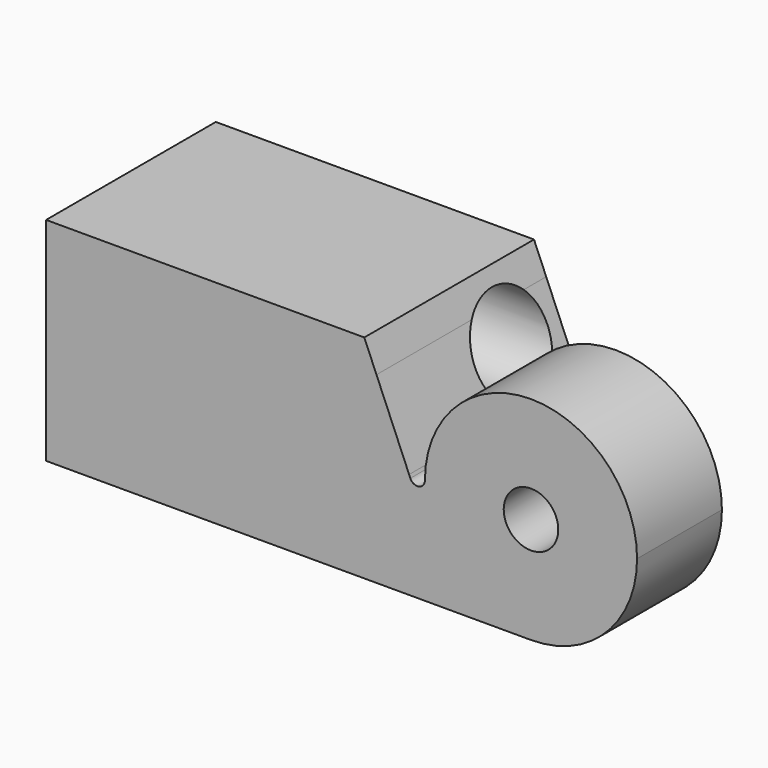
from build123d import *

# Parameters (mm, degrees)
F1_DEPTH       = 7
F2_D           = 3.6
F3_DEPTH       = 7
F5_D           = 3.5
F5_START       = 3.577541
F5_CBORE_D     = 6
F5_CBORE_DEPTH = 6


with BuildPart() as f1:
    # F0 (on Front) → F1 (new body)
    with BuildSketch(Plane.XZ):
        with BuildLine():
            Line((0, -7), (0, -1.45688))
            ThreePointArc((0, -1.45688), (-0.092433, -0.905477), (-0.1415, -0.348537))
            ThreePointArc((-0.1415, -0.348537), (-0.592364, -0.491395), (-0.960586, -0.194579))
            Line((-0.960586, -0.194579), (-1.042787, 0))
            Line((-1.042787, 0), (-3.195953, 5.096746))
            Line((-3.195953, 5.096746), (-4, 7))
            Line((-4, 7), (-25, 7))
            Line((-25, 7), (-25, -7))
            Line((-25, -7), (0, -7))
        make_face()
        with BuildLine():
            ThreePointArc((5.54312, -7), (1.944187, -5.055813), (0, -1.45688))
            Line((0, -1.45688), (0, -7))
            Line((0, -7), (5.54312, -7))
        make_face()
        with BuildLine():
            ThreePointArc((-0.1415, -0.348537), (-0.092433, -0.905477), (0, -1.45688))
            ThreePointArc((0, -1.45688), (1.944187, -5.055813), (5.54312, -7))
            Line((5.54312, -7), (7, -7))
            ThreePointArc((7, -7), (2.050253, -4.949747), (0, 0))
            ThreePointArc((0, 0), (-0.036724, -0.188082), (-0.1415, -0.348537))
        make_face()
        with BuildLine():
            ThreePointArc((14, 0), (7, 7), (0, 0))
            ThreePointArc((0, 0), (2.050253, -4.949747), (7, -7))
            ThreePointArc((7, -7), (11.949747, -4.949747), (14, 0))
        make_face()
    extrude(amount=F1_DEPTH)

    # F2 (through all)
    with Locations(Plane(origin=(0, 0, 0), x_dir=(1, 0, 0), z_dir=(0, 1, 0))):
        with Locations((7, 0)):
            Hole(F2_D / 2)

    # F0 (on Front) → F3 (join)
    with BuildSketch(Plane.XZ):
        with BuildLine():
            Line((0, -7), (0, -1.45688))
            ThreePointArc((0, -1.45688), (-0.092433, -0.905477), (-0.1415, -0.348537))
            ThreePointArc((-0.1415, -0.348537), (-0.592364, -0.491395), (-0.960586, -0.194579))
            Line((-0.960586, -0.194579), (-1.042787, 0))
            Line((-1.042787, 0), (-3.195953, 5.096746))
            Line((-3.195953, 5.096746), (-4, 7))
            Line((-4, 7), (-25, 7))
            Line((-25, 7), (-25, -7))
            Line((-25, -7), (0, -7))
        make_face()
        with BuildLine():
            ThreePointArc((5.54312, -7), (1.944187, -5.055813), (0, -1.45688))
            Line((0, -1.45688), (0, -7))
            Line((0, -7), (5.54312, -7))
        make_face()
    extrude(amount=-F3_DEPTH)

    # F5 (through all)
    # its depths count from where the whole tool has entered the part; down to there all is cleared
    with Locations(Plane.YZ.offset(-F5_START)):
        with Locations((3, 3)):
            CounterBoreHole(F5_D / 2, F5_CBORE_D / 2, F5_CBORE_DEPTH)


solid = f1.part
